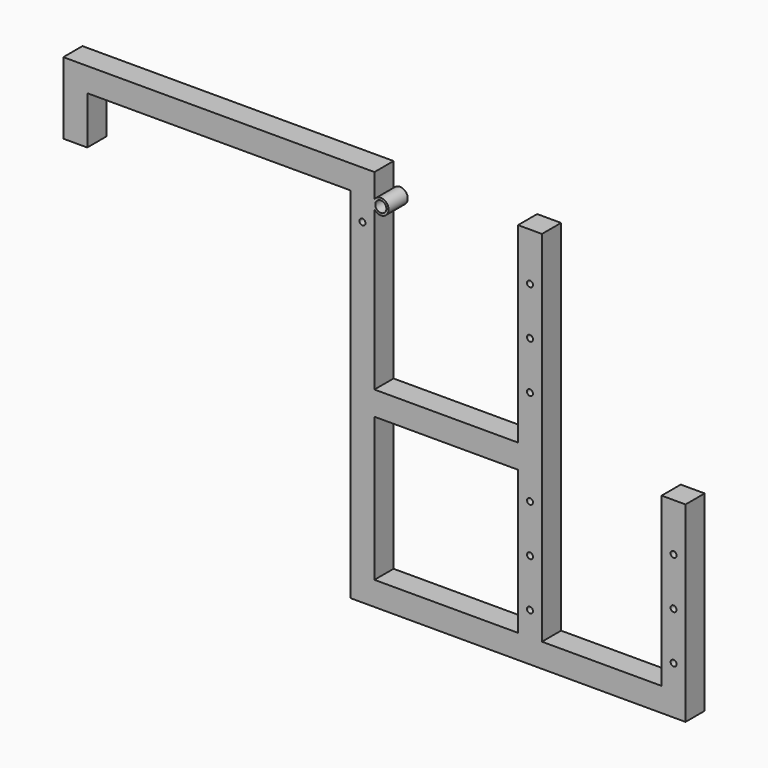
from build123d import *

# Parameters (mm, degrees)
F0_W      = 279.4
F0_H      = 25.4
F0_W_2    = 152.4
F0_W_3    = 25.4
F0_W_4    = 127
F1_DEPTH  = 12.7
F2_R      = 3.175
F3_DEPTH  = 50.8
F4_DEPTH  = 25.4
F5_R      = 8.255
F6_DEPTH  = 25.4
F9_R      = 5.8951712564
F10_DEPTH = 25.4


# Not quite as in the source:
# - the program builds the solid bodies; features that only make, move or delete a surface that nothing else refers to are left out


with BuildPart() as f1:
    # F0 (on Front) → F1 (new body, symmetric)
    with BuildSketch(Plane.XZ):
        with Locations((139.7, -12.7)):
            Rectangle(F0_W, F0_H)
        Polygon((0, -25.4), (0, 0), (-25.4, 0), (-25.4, -76.2), (0, -76.2), align=None)
        Polygon((304.8, 0), (279.4, 0), (279.4, -25.4), (279.4, -406.4), (304.8, -406.4), (304.8, -381), (304.8, -228.6), (304.8, -203.2), align=None)
        with Locations((381, -215.9)):
            Rectangle(F0_W_2, F0_H)
        with Locations((381, -393.7)):
            Rectangle(F0_W_2, F0_H)
        Polygon((457.2, 0), (457.2, -203.2), (457.2, -228.6), (457.2, -381), (482.6, -381), (482.6, 0), align=None)
        with Locations((469.9, -393.7)):
            Rectangle(F0_W_3, F0_H)
        with Locations((546.1, -393.7)):
            Rectangle(F0_W_4, F0_H)
        Polygon((609.6, -381), (609.6, -406.4), (635, -406.4), (635, -203.2), (609.6, -203.2), align=None)
    extrude(amount=F1_DEPTH, both=True)

    # F2 (on face) → F3 (cut)
    with BuildSketch(Plane.XZ.offset(12.7)):
        with Locations((469.9, -101.6)):
            Circle(F2_R)
        with Locations((469.9, -50.8)):
            Circle(F2_R)
        with Locations((469.9, -152.4)):
            Circle(F2_R)
        with Locations((469.9, -304.8)):
            Circle(F2_R)
        with Locations((469.9, -254)):
            Circle(F2_R)
        with Locations((469.9, -355.6)):
            Circle(F2_R)
        with Locations((622.3, -304.8)):
            Circle(F2_R)
        with Locations((622.3, -254)):
            Circle(F2_R)
        with Locations((622.3, -355.6)):
            Circle(F2_R)
        with Locations((292.1, -50.8)):
            Circle(F2_R)
    extrude(amount=F3_DEPTH, mode=Mode.SUBTRACT)

    # F2 (on face) → F4 (cut)
    with BuildSketch(Plane.XZ.offset(12.7)):
        with Locations((469.9, -101.6)):
            Circle(F2_R)
        with Locations((469.9, -50.8)):
            Circle(F2_R)
        with Locations((469.9, -152.4)):
            Circle(F2_R)
        with Locations((469.9, -304.8)):
            Circle(F2_R)
        with Locations((469.9, -254)):
            Circle(F2_R)
        with Locations((469.9, -355.6)):
            Circle(F2_R)
        with Locations((622.3, -304.8)):
            Circle(F2_R)
        with Locations((622.3, -254)):
            Circle(F2_R)
        with Locations((622.3, -355.6)):
            Circle(F2_R)
        with Locations((292.1, -50.8)):
            Circle(F2_R)
    extrude(amount=-F4_DEPTH, mode=Mode.SUBTRACT)

    # F5 (on face) → F6 (join)
    with BuildSketch(Plane.XZ.offset(12.7)):
        with Locations((311.5870648182, -30.0990186373)):
            Circle(F5_R)
    extrude(amount=-F6_DEPTH)

    # F9 (on face) → F10 (cut)
    with BuildSketch(Plane.XZ.offset(12.7)):
        with Locations((311.5870648182, -30.0990186373)):
            Circle(F9_R)
    extrude(amount=-F10_DEPTH, mode=Mode.SUBTRACT)


solid = f1.part
